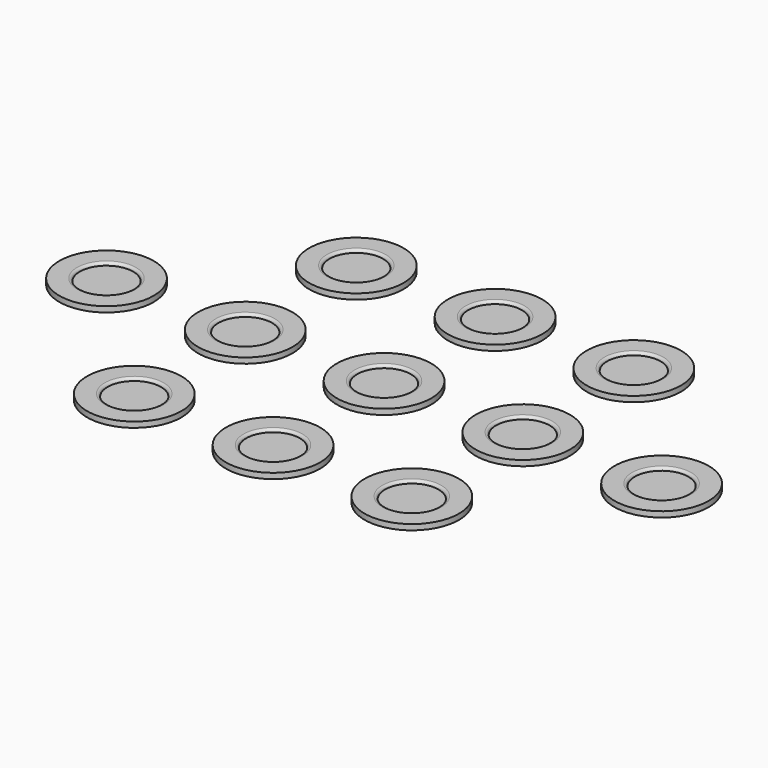
from build123d import *

# Parameters (mm, degrees)
F0_R     = 4.8895
F1_DEPTH = 0.508
F0_R_2   = 8.636
F2_DEPTH = 1.016
F3_R     = 0.50799


# Not quite as in the source:
# - a fillet or chamfer is up to 0.001 mm smaller than in the source, because OpenCascade refuses the exact size


with BuildPart() as f1:
    # F0 (on Top) → F1 (new body)
    with BuildSketch(Plane.XY):
        Circle(F0_R)
    extrude(amount=F1_DEPTH)

    # F0 (on Top) → F2 (join)
    with BuildSketch(Plane.XY):
        Circle(F0_R_2)
        Circle(F0_R, mode=Mode.SUBTRACT)
    extrude(amount=F2_DEPTH)

    # F3 (radius 0.508 in the source; OpenCascade refuses exactly that, so slightly less here)
    f3_edges = [f1.edges().sort_by_distance(p)[0] for p in [
        (-4.8895, 0, 1.016),
    ]]
    fillet(f3_edges, radius=F3_R)


with BuildPart() as f4_1:
    # F4: copy of F1
    add(f1.part.moved(Location((0, 25.4, 0))))


with BuildPart() as f5_1:
    # F5: copy of F1
    add(f1.part.moved(Location((0, -25.4, 0))))


with BuildPart() as f6_1:
    # F6: copy of F1
    add(f1.part.moved(Location((25.4, 0, 0))))


with BuildPart() as f7_1:
    # F7: copy of F1
    add(f1.part.moved(Location((-25.4, 0, 0))))


with BuildPart() as f8_1:
    # F8: copy of F6_1
    add(f6_1.part.moved(Location((25.4, 0, 0))))


with BuildPart() as f9_1:
    # F9: copy of F7_1
    add(f7_1.part.moved(Location((-25.4, 0, 0))))


with BuildPart() as f10_1:
    # F10: copy of F7_1
    add(f7_1.part.moved(Location((0, -25.4, 0))))


with BuildPart() as f11_1:
    # F11: copy of F7_1
    add(f7_1.part.moved(Location((0, 25.4, 0))))


with BuildPart() as f12_1:
    # F12: copy of F6_1
    add(f6_1.part.moved(Location((0, -25.4, 0))))


with BuildPart() as f13_1:
    # F13: copy of F6_1
    add(f6_1.part.moved(Location((0, 25.4, 0))))


solid = Compound([f1.part, f4_1.part, f5_1.part, f6_1.part, f7_1.part, f8_1.part, f9_1.part, f10_1.part, f11_1.part, f12_1.part, f13_1.part])
